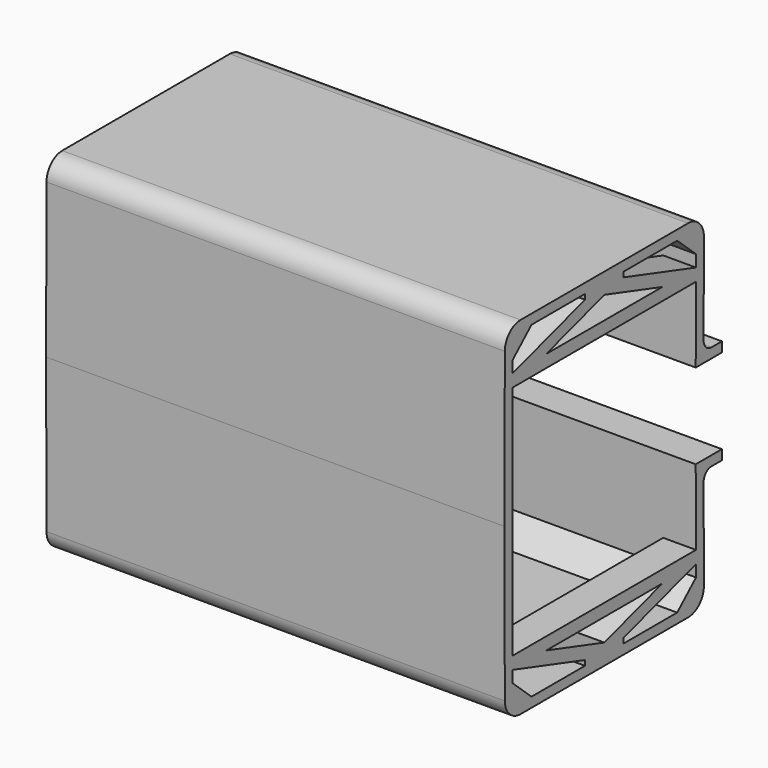
from build123d import *

# Parameters (mm, degrees)
F1_DEPTH = 70
F3_DEPTH = 10


# Not quite as in the source:
# - a feature names something its author has since deleted; it is built from what else it names


with BuildPart() as f1:
    # F0 (on Right) → F1 (new body)
    with BuildSketch(Plane.YZ):
        with BuildLine():
            Line((35.0004041982, -43.4744954109), (27.8094485444, -50))
            Line((27.8094485444, -50), (-27.8090443462, -50))
            Line((-27.8090443462, -50), (-35, -43.4744954109))
            Line((-35, -43.4744954109), (-35.1477400841, 0))
            Line((-35.1477400841, 0), (-38.1477574069, 0))
            Line((-38.1477574069, 0), (-37.988001967, -47.0101745328))
            ThreePointArc((-37.988001967, -47.0101745328), (-36.2312971095, -51.2420067187), (-32, -53))
            Line((-32, -53), (32, -53))
            ThreePointArc((32, -53), (36.3403848268, -51.1600325097), (38.0115591918, -46.7519039894))
            Line((38.0115591918, -46.7519039894), (37.917284091, -19.0101948899))
            ThreePointArc((37.917284091, -19.0101948899), (38.792345044, -16.8822871618), (40.9172667684, -16))
            Line((40.9172667684, -16), (44.8968422253, -16))
            Line((44.8968422253, -16), (44.8968422253, -13))
            Line((44.8968422253, -13), (34.8968422253, -13))
            Line((34.8968422253, -13), (35.0004041982, -43.4744954109))
        make_face()
    extrude(amount=F1_DEPTH)

    # F2 (on face) → F3 (join)
    with BuildSketch(Plane.YZ.offset(70)):
        Polygon((34.9751985597, -36.0573992247), (-35.0252056385, -36.0573992247), (-35.0122565756, -39.8678341294), (-7.3888426073, -48.4471021518), (-7.3888426073, -50), (-2.3888426073, -50), (2.3879472654, -50), (7.3879472654, -50), (7.3879472654, -48.4459963804), (34.9881476226, -39.8678341294), align=None)
        Polygon((0, -46.7519039894), (-22.1652372944, -39.8678341294), (22.1494653338, -39.8678341294), align=None, mode=Mode.SUBTRACT)
    extrude(amount=-F3_DEPTH)

    # F4: F1 across plane


with BuildPart() as f1_1:
    add(f1.part)
    add(f1.part.mirror(Plane.YZ))

    # F5: F1 across plane


with BuildPart() as f1_2:
    add(f1_1.part)
    add(f1_1.part.mirror(Plane.XY))


solid = f1_2.part
